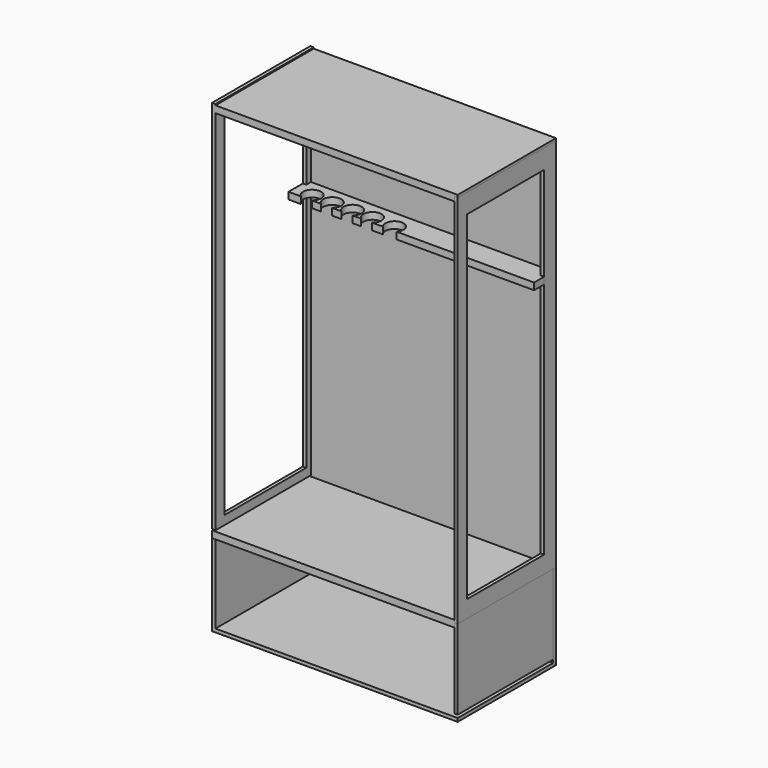
from build123d import *

# Parameters (mm, degrees)
F0_W      = 914.4
F0_H      = 457.2
F1_DEPTH  = 12.7
F2_W      = 457.2
F2_H      = 304.8
F3_DEPTH  = 12.7
F5_W      = 457.2
F5_H      = 304.8
F6_DEPTH  = 12.7
F8_W      = 913.9710068703
F8_H      = 456.640124321
F9_DEPTH  = 25.4
F10_W     = 914.4
F10_H     = 1701.8
F11_DEPTH = 12.7
F13_W     = 914.4
F13_H     = 457.2
F14_DEPTH = 25.4
F15_W     = 457.2
F15_H     = 1397
F16_DEPTH = 12.7
F17_W     = 357.7546179295
F17_H     = 1261.1754238605
F18_DEPTH = 914.401
F19_W     = 457.2
F19_H     = 1397
F20_DEPTH = 12.7
F21_W     = 380.351215601
F21_H     = 1307.6837956905
F22_DEPTH = 914.401
F24_W     = 914.4
F24_H     = 101.6
F25_DEPTH = 25.4
F27_DEPTH = 25.4
F29_DEPTH = 25.4
F31_DEPTH = 25.4
F33_DEPTH = 25.4
F35_DEPTH = 25.4


# Not quite as in the source:
# - ends of sketch curves that miss each other by under 0.0002 mm in the source are joined


with BuildPart() as f1:
    # F0 (on Top) → F1 (new body)
    with BuildSketch(Plane.XY):
        with Locations((457.2, -228.6)):
            Rectangle(F0_W, F0_H)
    extrude(amount=F1_DEPTH)

    # F2 (on Right) → F3 (join)
    with BuildSketch(Plane.YZ):
        with Locations((-228.6, 152.4)):
            Rectangle(F2_W, F2_H)
    extrude(amount=F3_DEPTH)

    # F8 (on offset) → F9 (join)
    with BuildSketch(Plane.XY.offset(304.8)):
        with Locations((456.9855034351, -228.3200621605)):
            Rectangle(F8_W, F8_H)
    extrude(amount=F9_DEPTH)


with BuildPart() as f6:
    # F5 (on offset) → F6 (new body)
    with BuildSketch(Plane.YZ.offset(914.4)):
        with Locations((-228.6, 176.0915509423)):
            Rectangle(F5_W, F5_H)
    extrude(amount=-F6_DEPTH)


with BuildPart() as f11:
    # F10 (on Front) → F11 (new body)
    with BuildSketch(Plane.XZ):
        with Locations((457.2, 855.7587931213)):
            Rectangle(F10_W, F10_H)
    extrude(amount=F11_DEPTH)

    # F13 (on offset) → F14 (join)
    with BuildSketch(Plane.XY.offset(1701.8)):
        with Locations((457.2, -228.6)):
            Rectangle(F13_W, F13_H)
    extrude(amount=F14_DEPTH)

    # F19 (on Right) → F20 (join)
    with BuildSketch(Plane.YZ):
        with Locations((-228.6, 1033.0463655774)):
            Rectangle(F19_W, F19_H)
    extrude(amount=F20_DEPTH)

    # F21 (on Right) → F22 (cut, through all)
    with BuildSketch(Plane.YZ):
        with Locations((-224.9127179384, 1021.4712172747)):
            Rectangle(F21_W, F21_H)
    extrude(amount=F22_DEPTH, mode=Mode.SUBTRACT)

    # F24 (on offset) → F25 (join)
    with BuildSketch(Plane.XY.offset(1270)):
        with Locations((457.2, -50.8)):
            Rectangle(F24_W, F24_H)
    extrude(amount=F25_DEPTH)

    # F26 (on face) → F27 (cut)
    with BuildSketch(Plane.XY.offset(1295.4)):
        with BuildLine():
            Line((46.2475046515, -101.6), (86.683191359, -101.6))
            ThreePointArc((86.683191359, -101.6), (66.4653480053, -41.0647853812), (46.2475046515, -101.6))
        make_face()
    extrude(amount=-F27_DEPTH, mode=Mode.SUBTRACT)

    # F28 (on face) → F29 (cut)
    with BuildSketch(Plane.XY.offset(1295.4)):
        with BuildLine():
            Line((121.2305128574, -101.6), (161.6661995649, -101.6))
            ThreePointArc((161.6661995649, -101.6), (141.4483562112, -41.0647853812), (121.2305128574, -101.6))
        make_face()
    extrude(amount=-F29_DEPTH, mode=Mode.SUBTRACT)

    # F30 (on face) → F31 (cut)
    with BuildSketch(Plane.XY.offset(1295.4)):
        with BuildLine():
            Line((197.0332803288, -101.6), (238.13604395, -101.6))
            ThreePointArc((238.13604395, -101.6), (217.5846621394, -41.3188191494), (197.0332803288, -101.6))
        make_face()
    extrude(amount=-F31_DEPTH, mode=Mode.SUBTRACT)

    # F32 (on face) → F33 (cut)
    with BuildSketch(Plane.XY.offset(1295.4)):
        with BuildLine():
            Line((270.8255052567, -101.6), (311.2611919641, -101.6))
            ThreePointArc((311.2611919641, -101.6), (291.0433486104, -41.0647841533), (270.8255052567, -101.6))
        make_face()
    extrude(amount=-F33_DEPTH, mode=Mode.SUBTRACT)

    # F34 (on face) → F35 (cut)
    with BuildSketch(Plane.XY.offset(1295.4)):
        with BuildLine():
            Line((351.1739761807, -101.6), (403.0564038776, -101.6))
            ThreePointArc((403.0564038776, -101.6), (377.1151900291, -46.5327916681), (351.1739761807, -101.6))
        make_face()
    extrude(amount=-F35_DEPTH, mode=Mode.SUBTRACT)


with BuildPart() as f16:
    # F15 (on offset) → F16 (new body)
    with BuildSketch(Plane.YZ.offset(914.4)):
        with Locations((-228.6, 1019.5414156894)):
            Rectangle(F15_W, F15_H)
    extrude(amount=-F16_DEPTH)

    # F17 (on offset) → F18 (cut, through all)
    with BuildSketch(Plane.YZ.offset(914.4)):
        with Locations((-233.8642030954, 1015.2183622122)):
            Rectangle(F17_W, F17_H)
    extrude(amount=-F18_DEPTH, mode=Mode.SUBTRACT)


solid = Compound([f1.part, f6.part, f11.part, f16.part])
